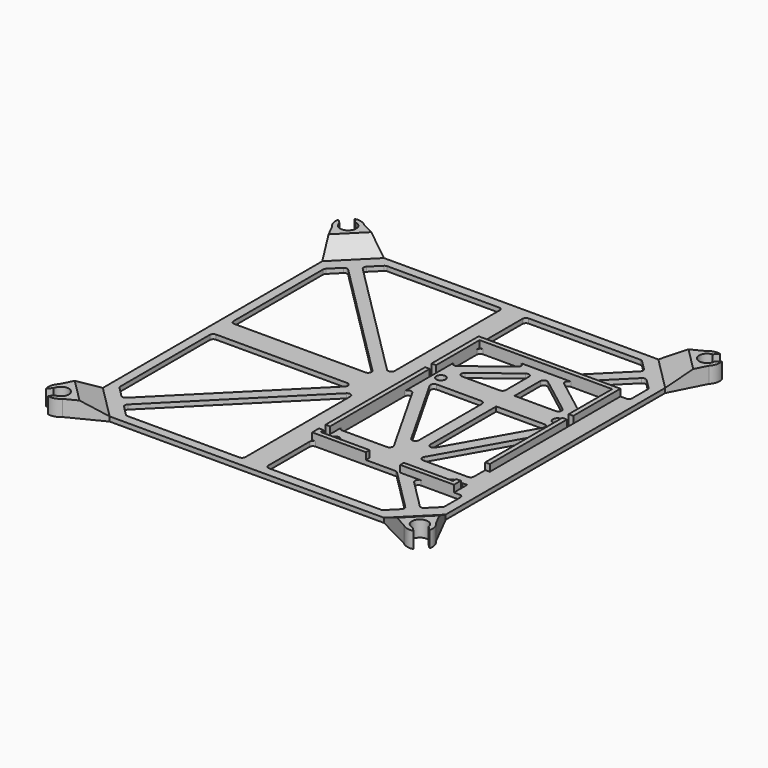
from build123d import *

# Parameters (mm, degrees)
F0_W          = 150
F0_H          = 150
F1_DEPTH      = 2
F2_W          = 62
F2_H          = 91
F2_W_2        = 58
F2_H_2        = 87
F3_DEPTH      = 3
F4_W          = 15
F4_H          = 2
F4_W_2        = 2
F4_H_2        = 14
F5_DEPTH      = 3
F6_R          = 2
F6_W          = 2
F6_H          = 3.5
F7_DEPTH      = 25
F9_DEPTH      = 5
F9_DEPTH_BACK = 2
F10_DEPTH     = 5
F11_DEPTH     = 5
F12_SIZE2     = 4.99999
F12_SIZE      = 9.99999
F12_2_SIZE2   = 4.99999
F12_2_SIZE    = 9.99999
F12_3_SIZE2   = 4.99999
F12_3_SIZE    = 9.99999
F12_4_SIZE2   = 4.99999
F12_4_SIZE    = 9.99999
F14_DEPTH     = 25
F16_DEPTH     = 25
F17_R         = 1.5
F18_R         = 1.5
F19_R         = 1.5
F20_R         = 1.5


# Not quite as in the source:
# - a fillet or chamfer is up to 0.001 mm smaller than in the source, because OpenCascade refuses the exact size


with BuildPart() as f1:
    # F0 (on Top) → F1 (new body)
    with BuildSketch(Plane.XY):
        Rectangle(F0_W, F0_H)
    extrude(amount=F1_DEPTH)

    # F2 (on face) → F3 (join)
    with BuildSketch(Plane.XY.offset(2)):
        with Locations((36, 0)):
            Rectangle(F2_W, F2_H)
        with Locations((36, 0)):
            Rectangle(F2_W_2, F2_H_2, mode=Mode.SUBTRACT)
    extrude(amount=F3_DEPTH)

    # F4 (on face) → F5 (cut)
    with BuildSketch(Plane.XY.offset(5)):
        with Locations((36, -44.5)):
            Rectangle(F4_W, F4_H)
        with Locations((66, -32.9)):
            Rectangle(F4_W_2, F4_H_2)
    extrude(amount=-F5_DEPTH, mode=Mode.SUBTRACT)

    # F6 (on face) → F7 (cut)
    with BuildSketch(Plane.XY.offset(5)):
        with Locations((61.5, -40)):
            Circle(F6_R)
        with Locations((61.5, 18)):
            Circle(F6_R)
        with Locations((66, -40)):
            Rectangle(F6_W, F6_H)
        with Locations((66, 18)):
            Rectangle(F6_W, F6_H)
        with Locations((6, -40)):
            Rectangle(F6_W, F6_H)
        with Locations((6, 18)):
            Rectangle(F6_W, F6_H)
        with Locations((10.5, 18)):
            Circle(F6_R)
        with Locations((10.5, -40)):
            Circle(F6_R)
    extrude(amount=-F7_DEPTH, mode=Mode.SUBTRACT)

    # F8 (on face) → F9 (join, two sides)
    with BuildSketch(Plane.XY.offset(2)) as f9_sk:
        with BuildLine():
            ThreePointArc((82.0110086434, 78.1219213469), (76.0606601718, 76.0606601718), (78.1219213469, 82.0110086434))
            Line((78.1219213469, 82.0110086434), (79.959038654, 83.8481259505))
            ThreePointArc((79.959038654, 83.8481259505), (77.1120291579, 83.8481259505), (74.6464466094, 82.4246212025))
            Line((74.6464466094, 82.4246212025), (60, 75))
            Line((60, 75), (75, 60))
            Line((75, 60), (82.4246212025, 74.6464466094))
            ThreePointArc((82.4246212025, 74.6464466094), (83.8481259505, 77.1120291579), (83.8481259505, 79.959038654))
            Line((83.8481259505, 79.959038654), (82.0110086434, 78.1219213469))
        make_face()
        with BuildLine():
            Line((-60, 75), (-74.6464466094, 82.4246212025))
            ThreePointArc((-74.6464466094, 82.4246212025), (-77.1120291579, 83.8481259505), (-79.959038654, 83.8481259505))
            Line((-79.959038654, 83.8481259505), (-78.1219213469, 82.0110086434))
            ThreePointArc((-78.1219213469, 82.0110086434), (-76.0606601718, 76.0606601718), (-82.0110086434, 78.1219213469))
            Line((-82.0110086434, 78.1219213469), (-83.8481259505, 79.959038654))
            ThreePointArc((-83.8481259505, 79.959038654), (-83.8481259505, 77.1120291579), (-82.4246212025, 74.6464466094))
            Line((-82.4246212025, 74.6464466094), (-75, 60))
            Line((-75, 60), (-60, 75))
        make_face()
        with BuildLine():
            Line((-75, -60), (-82.4246212025, -74.6464466094))
            ThreePointArc((-82.4246212025, -74.6464466094), (-83.8481259505, -77.1120291579), (-83.8481259505, -79.959038654))
            Line((-83.8481259505, -79.959038654), (-82.0110086434, -78.1219213469))
            ThreePointArc((-82.0110086434, -78.1219213469), (-76.0606601718, -76.0606601718), (-78.1219213469, -82.0110086434))
            Line((-78.1219213469, -82.0110086434), (-79.959038654, -83.8481259505))
            ThreePointArc((-79.959038654, -83.8481259505), (-77.1120291579, -83.8481259505), (-74.6464466094, -82.4246212025))
            Line((-74.6464466094, -82.4246212025), (-60, -75))
            Line((-60, -75), (-75, -60))
        make_face()
        with BuildLine():
            Line((60, -75), (74.6464466094, -82.4246212025))
            ThreePointArc((74.6464466094, -82.4246212025), (77.1120291579, -83.8481259505), (79.959038654, -83.8481259505))
            Line((79.959038654, -83.8481259505), (78.1219213469, -82.0110086434))
            ThreePointArc((78.1219213469, -82.0110086434), (76.0606601718, -76.0606601718), (82.0110086434, -78.1219213469))
            Line((82.0110086434, -78.1219213469), (83.8481259505, -79.959038654))
            ThreePointArc((83.8481259505, -79.959038654), (83.8481259505, -77.1120291579), (82.4246212025, -74.6464466094))
            Line((82.4246212025, -74.6464466094), (75, -60))
            Line((75, -60), (60, -75))
        make_face()
    extrude(amount=F9_DEPTH)
    extrude(f9_sk.sketch, amount=-F9_DEPTH_BACK)

    # F8 (on face) → F10 (join)
    with BuildSketch(Plane.XY.offset(2)):
        with BuildLine():
            ThreePointArc((82.0110086434, 78.1219213469), (76.0606601718, 76.0606601718), (78.1219213469, 82.0110086434))
            Line((78.1219213469, 82.0110086434), (79.959038654, 83.8481259505))
            ThreePointArc((79.959038654, 83.8481259505), (77.1120291579, 83.8481259505), (74.6464466094, 82.4246212025))
            Line((74.6464466094, 82.4246212025), (60, 75))
            Line((60, 75), (75, 60))
            Line((75, 60), (82.4246212025, 74.6464466094))
            ThreePointArc((82.4246212025, 74.6464466094), (83.8481259505, 77.1120291579), (83.8481259505, 79.959038654))
            Line((83.8481259505, 79.959038654), (82.0110086434, 78.1219213469))
        make_face()
        with BuildLine():
            Line((-60, 75), (-74.6464466094, 82.4246212025))
            ThreePointArc((-74.6464466094, 82.4246212025), (-77.1120291579, 83.8481259505), (-79.959038654, 83.8481259505))
            Line((-79.959038654, 83.8481259505), (-78.1219213469, 82.0110086434))
            ThreePointArc((-78.1219213469, 82.0110086434), (-76.0606601718, 76.0606601718), (-82.0110086434, 78.1219213469))
            Line((-82.0110086434, 78.1219213469), (-83.8481259505, 79.959038654))
            ThreePointArc((-83.8481259505, 79.959038654), (-83.8481259505, 77.1120291579), (-82.4246212025, 74.6464466094))
            Line((-82.4246212025, 74.6464466094), (-75, 60))
            Line((-75, 60), (-60, 75))
        make_face()
        with BuildLine():
            Line((-75, -60), (-82.4246212025, -74.6464466094))
            ThreePointArc((-82.4246212025, -74.6464466094), (-83.8481259505, -77.1120291579), (-83.8481259505, -79.959038654))
            Line((-83.8481259505, -79.959038654), (-82.0110086434, -78.1219213469))
            ThreePointArc((-82.0110086434, -78.1219213469), (-76.0606601718, -76.0606601718), (-78.1219213469, -82.0110086434))
            Line((-78.1219213469, -82.0110086434), (-79.959038654, -83.8481259505))
            ThreePointArc((-79.959038654, -83.8481259505), (-77.1120291579, -83.8481259505), (-74.6464466094, -82.4246212025))
            Line((-74.6464466094, -82.4246212025), (-60, -75))
            Line((-60, -75), (-75, -60))
        make_face()
        with BuildLine():
            Line((60, -75), (74.6464466094, -82.4246212025))
            ThreePointArc((74.6464466094, -82.4246212025), (77.1120291579, -83.8481259505), (79.959038654, -83.8481259505))
            Line((79.959038654, -83.8481259505), (78.1219213469, -82.0110086434))
            ThreePointArc((78.1219213469, -82.0110086434), (76.0606601718, -76.0606601718), (82.0110086434, -78.1219213469))
            Line((82.0110086434, -78.1219213469), (83.8481259505, -79.959038654))
            ThreePointArc((83.8481259505, -79.959038654), (83.8481259505, -77.1120291579), (82.4246212025, -74.6464466094))
            Line((82.4246212025, -74.6464466094), (75, -60))
            Line((75, -60), (60, -75))
        make_face()
    extrude(amount=F10_DEPTH)

    # F8 (on face) → F11 (join)
    with BuildSketch(Plane.XY.offset(2)):
        with BuildLine():
            ThreePointArc((82.0110086434, 78.1219213469), (76.0606601718, 76.0606601718), (78.1219213469, 82.0110086434))
            Line((78.1219213469, 82.0110086434), (79.959038654, 83.8481259505))
            ThreePointArc((79.959038654, 83.8481259505), (77.1120291579, 83.8481259505), (74.6464466094, 82.4246212025))
            Line((74.6464466094, 82.4246212025), (60, 75))
            Line((60, 75), (75, 60))
            Line((75, 60), (82.4246212025, 74.6464466094))
            ThreePointArc((82.4246212025, 74.6464466094), (83.8481259505, 77.1120291579), (83.8481259505, 79.959038654))
            Line((83.8481259505, 79.959038654), (82.0110086434, 78.1219213469))
        make_face()
        with BuildLine():
            Line((-60, 75), (-74.6464466094, 82.4246212025))
            ThreePointArc((-74.6464466094, 82.4246212025), (-77.1120291579, 83.8481259505), (-79.959038654, 83.8481259505))
            Line((-79.959038654, 83.8481259505), (-78.1219213469, 82.0110086434))
            ThreePointArc((-78.1219213469, 82.0110086434), (-76.0606601718, 76.0606601718), (-82.0110086434, 78.1219213469))
            Line((-82.0110086434, 78.1219213469), (-83.8481259505, 79.959038654))
            ThreePointArc((-83.8481259505, 79.959038654), (-83.8481259505, 77.1120291579), (-82.4246212025, 74.6464466094))
            Line((-82.4246212025, 74.6464466094), (-75, 60))
            Line((-75, 60), (-60, 75))
        make_face()
        with BuildLine():
            Line((-75, -60), (-82.4246212025, -74.6464466094))
            ThreePointArc((-82.4246212025, -74.6464466094), (-83.8481259505, -77.1120291579), (-83.8481259505, -79.959038654))
            Line((-83.8481259505, -79.959038654), (-82.0110086434, -78.1219213469))
            ThreePointArc((-82.0110086434, -78.1219213469), (-76.0606601718, -76.0606601718), (-78.1219213469, -82.0110086434))
            Line((-78.1219213469, -82.0110086434), (-79.959038654, -83.8481259505))
            ThreePointArc((-79.959038654, -83.8481259505), (-77.1120291579, -83.8481259505), (-74.6464466094, -82.4246212025))
            Line((-74.6464466094, -82.4246212025), (-60, -75))
            Line((-60, -75), (-75, -60))
        make_face()
        with BuildLine():
            Line((60, -75), (74.6464466094, -82.4246212025))
            ThreePointArc((74.6464466094, -82.4246212025), (77.1120291579, -83.8481259505), (79.959038654, -83.8481259505))
            Line((79.959038654, -83.8481259505), (78.1219213469, -82.0110086434))
            ThreePointArc((78.1219213469, -82.0110086434), (76.0606601718, -76.0606601718), (82.0110086434, -78.1219213469))
            Line((82.0110086434, -78.1219213469), (83.8481259505, -79.959038654))
            ThreePointArc((83.8481259505, -79.959038654), (83.8481259505, -77.1120291579), (82.4246212025, -74.6464466094))
            Line((82.4246212025, -74.6464466094), (75, -60))
            Line((75, -60), (60, -75))
        make_face()
    extrude(amount=F11_DEPTH)

    # F12 (size 10 and 5 in the source; OpenCascade refuses exactly that, so slightly less here)
    f12_edges = [f1.edges().sort_by_distance(p)[0] for p in [
        (-67.5, 67.5, 7),
    ]]
    f12_side = f1.faces().sort_by_distance((-72.538706, 72.538706, 7))[0]
    chamfer(f12_edges, length=F12_SIZE, length2=F12_SIZE2, reference=f12_side)

    # F12#2 (size 10 and 5 in the source; OpenCascade refuses exactly that, so slightly less here)
    f12_2_edges = [f1.edges().sort_by_distance(p)[0] for p in [
        (67.5, 67.5, 7),
    ]]
    f12_2_side = f1.faces().sort_by_distance((72.538706, 72.538706, 7))[0]
    chamfer(f12_2_edges, length=F12_2_SIZE, length2=F12_2_SIZE2, reference=f12_2_side)

    # F12#3 (size 10 and 5 in the source; OpenCascade refuses exactly that, so slightly less here)
    f12_3_edges = [f1.edges().sort_by_distance(p)[0] for p in [
        (67.5, -67.5, 7),
    ]]
    f12_3_side = f1.faces().sort_by_distance((72.538706, -72.538706, 7))[0]
    chamfer(f12_3_edges, length=F12_3_SIZE, length2=F12_3_SIZE2, reference=f12_3_side)

    # F12#4 (size 10 and 5 in the source; OpenCascade refuses exactly that, so slightly less here)
    f12_4_edges = [f1.edges().sort_by_distance(p)[0] for p in [
        (-67.5, -67.5, 7),
    ]]
    f12_4_side = f1.faces().sort_by_distance((-72.538706, -72.538706, 7))[0]
    chamfer(f12_4_edges, length=F12_4_SIZE, length2=F12_4_SIZE2, reference=f12_4_side)

    # F13 (on face) → F14 (cut)
    with BuildSketch(Plane.XY.offset(2)):
        Polygon((-65.267766953, 61.732233047), (-71, 56), (-71, 5), (-8.5355339059, 5), align=None)
        with BuildLine():
            ThreePointArc((-7.5606601718, 11.0961940777), (-5.9259748515, 10.7710349507), (-5, 12.1568542495))
            Line((-5, 12.1568542495), (-5, 71))
            Line((-5, 71), (-56, 71))
            Line((-56, 71), (-60.6715728753, 66.3284271247))
            ThreePointArc((-60.6715728753, 66.3284271247), (-61.1109127035, 65.267766953), (-60.6715728753, 64.2071067812))
            Line((-60.6715728753, 64.2071067812), (-7.5606601718, 11.0961940777))
        make_face()
        Polygon((-5, -71), (-5, -8.5355339059), (-61.732233047, -65.267766953), (-56, -71), align=None)
        Polygon((-8.5355339059, -5), (-71, -5), (-71, -56), (-65.267766953, -61.732233047), align=None)
        Polygon((56, 71), (5, 71), (5, 45.5), (41.9644660941, 45.5), (61.732233047, 65.267766953), align=None)
        Polygon((41.9644660941, -45.5), (5, -45.5), (5, -71), (56, -71), (61.732233047, -65.267766953), align=None)
        Polygon((71, 56), (65.267766953, 61.732233047), (49.0355339059, 45.5), (71, 45.5), align=None)
        Polygon((71, -45.5), (49.0355339059, -45.5), (65.267766953, -61.732233047), (71, -56), align=None)
    extrude(amount=-F14_DEPTH, mode=Mode.SUBTRACT)

    # F15 (on face) → F16 (cut)
    with BuildSketch(Plane.XY.offset(5)):
        with BuildLine():
            ThreePointArc((40.9107577546, 38.5114634802), (39.3352205749, 38.6642519615), (38.5, 37.3196076531))
            Line((38.5, 37.3196076531), (38.5, 24.75))
            ThreePointArc((38.5, 24.75), (38.9393398282, 23.6893398282), (40, 23.25))
            Line((40, 23.25), (56.449116188, 23.25))
            ThreePointArc((56.449116188, 23.25), (57.8699933362, 24.2692629308), (57.3598739427, 25.941855827))
            Line((57.3598739427, 25.941855827), (40.9107577546, 38.5114634802))
        make_face()
        with BuildLine():
            ThreePointArc((40, 23.25), (38.9393398282, 23.6893398282), (38.5, 24.75))
            Line((38.5, 24.75), (38.5, 23.25))
            Line((38.5, 23.25), (40, 23.25))
        make_face()
        with BuildLine():
            ThreePointArc((7, -32), (7.4393398282, -33.0606601718), (8.5, -33.5))
            Line((8.5, -33.5), (28.0517971478, -33.5))
            ThreePointArc((28.0517971478, -33.5), (29.3478570196, -32.7551349607), (29.3567306415, -31.2603050784))
            Line((29.3567306415, -31.2603050784), (9.8049334937, 3.232016305))
            ThreePointArc((9.8049334937, 3.232016305), (8.1175083273, 3.9427351589), (7, 2.4923213834))
            Line((7, 2.4923213834), (7, -32))
        make_face()
        with BuildLine():
            Line((33.5, -22.7423213834), (33.5, 11.75))
            ThreePointArc((33.5, 11.75), (33.0606601718, 12.8106601718), (32, 13.25))
            Line((32, 13.25), (12.4482028522, 13.25))
            ThreePointArc((12.4482028522, 13.25), (11.1521429804, 12.5051349607), (11.1432693585, 11.0103050784))
            Line((11.1432693585, 11.0103050784), (30.6950665063, -23.482016305))
            ThreePointArc((30.6950665063, -23.482016305), (32.3824916727, -24.1927351589), (33.5, -22.7423213834))
        make_face()
        with BuildLine():
            Line((40, 13.25), (38.5, 13.25))
            Line((38.5, 13.25), (38.5, 11.75))
            ThreePointArc((38.5, 11.75), (38.9393398282, 12.8106601718), (40, 13.25))
        make_face()
        with BuildLine():
            ThreePointArc((42.6432693585, -31.2603050784), (42.6521429804, -32.7551349607), (43.9482028522, -33.5))
            Line((43.9482028522, -33.5), (63.5, -33.5))
            ThreePointArc((63.5, -33.5), (64.5606601718, -33.0606601718), (65, -32))
            Line((65, -32), (65, 2.4923213834))
            ThreePointArc((65, 2.4923213834), (63.8824916727, 3.9427351589), (62.1950665063, 3.232016305))
            Line((62.1950665063, 3.232016305), (42.6432693585, -31.2603050784))
        make_face()
        with BuildLine():
            ThreePointArc((40, 13.25), (38.9393398282, 12.8106601718), (38.5, 11.75))
            Line((38.5, 11.75), (38.5, -22.7423213834))
            ThreePointArc((38.5, -22.7423213834), (39.6175083273, -24.1927351589), (41.3049334937, -23.482016305))
            Line((41.3049334937, -23.482016305), (60.8567306415, 11.0103050784))
            ThreePointArc((60.8567306415, 11.0103050784), (60.8478570196, 12.5051349607), (59.5517971478, 13.25))
            Line((59.5517971478, 13.25), (40, 13.25))
        make_face()
        with BuildLine():
            ThreePointArc((33.5, 37.3196076531), (32.6647794251, 38.6642519615), (31.0892422454, 38.5114634802))
            Line((31.0892422454, 38.5114634802), (14.6401260573, 25.941855827))
            ThreePointArc((14.6401260573, 25.941855827), (14.1300066638, 24.2692629308), (15.550883812, 23.25))
            Line((15.550883812, 23.25), (32, 23.25))
            ThreePointArc((32, 23.25), (33.0606601718, 23.6893398282), (33.5, 24.75))
            Line((33.5, 24.75), (33.5, 37.3196076531))
        make_face()
        with BuildLine():
            Line((7, 42), (7, 29.4303923469))
            ThreePointArc((7, 29.4303923469), (7.8352205749, 28.0857480385), (9.4107577546, 28.2385365198))
            Line((9.4107577546, 28.2385365198), (25.8598739427, 40.808144173))
            ThreePointArc((25.8598739427, 40.808144173), (26.3699933362, 42.4807370692), (24.949116188, 43.5))
            Line((24.949116188, 43.5), (8.5, 43.5))
            ThreePointArc((8.5, 43.5), (7.4393398282, 43.0606601718), (7, 42))
        make_face()
        with BuildLine():
            ThreePointArc((47.050883812, 43.5), (45.6300066638, 42.4807370692), (46.1401260573, 40.808144173))
            Line((46.1401260573, 40.808144173), (62.5892422454, 28.2385365198))
            ThreePointArc((62.5892422454, 28.2385365198), (64.1647794251, 28.0857480385), (65, 29.4303923469))
            Line((65, 29.4303923469), (65, 42))
            ThreePointArc((65, 42), (64.5606601718, 43.0606601718), (63.5, 43.5))
            Line((63.5, 43.5), (47.050883812, 43.5))
        make_face()
    extrude(amount=-F16_DEPTH, mode=Mode.SUBTRACT)

    # F17
    f17_edges = [f1.edges().sort_by_distance(p)[0] for p in [
        (-56, 71, 1),
    ]]
    fillet(f17_edges, radius=F17_R)

    # F18
    f18_edges = [f1.edges().sort_by_distance(p)[0] for p in [
        (-5, 71, 1),
        (-8.535534, 5, 1),
        (-71, 5, 1),
        (-65.267767, 61.732233, 1),
        (-71, 56, 1),
    ]]
    fillet(f18_edges, radius=F18_R)

    # F19
    f19_edges = [f1.edges().sort_by_distance(p)[0] for p in [
        (-5, -8.535534, 1),
        (-8.535534, -5, 1),
        (-71, -5, 1),
        (-71, -56, 1),
        (-61.732233, -65.267767, 1),
        (-65.267767, -61.732233, 1),
        (-56, -71, 1),
        (-5, -71, 1),
        (5, -71, 1),
        (5, -45.5, 1),
        (49.035534, -45.5, 1),
        (41.964466, -45.5, 1),
        (71, -45.5, 1),
        (71, -56, 1),
        (65.267767, -61.732233, 1),
        (65.267767, 61.732233, 1),
        (56, 71, 1),
        (61.732233, 65.267767, 1),
        (71, 56, 1),
        (71, 45.5, 1),
        (49.035534, 45.5, 1),
        (41.964466, 45.5, 1),
        (5, 45.5, 1),
        (5, 71, 1),
    ]]
    fillet(f19_edges, radius=F19_R)

    # F20
    f20_edges = [f1.edges().sort_by_distance(p)[0] for p in [
        (56, -71, 1),
        (61.732233, -65.267767, 1),
    ]]
    fillet(f20_edges, radius=F20_R)


solid = f1.part
